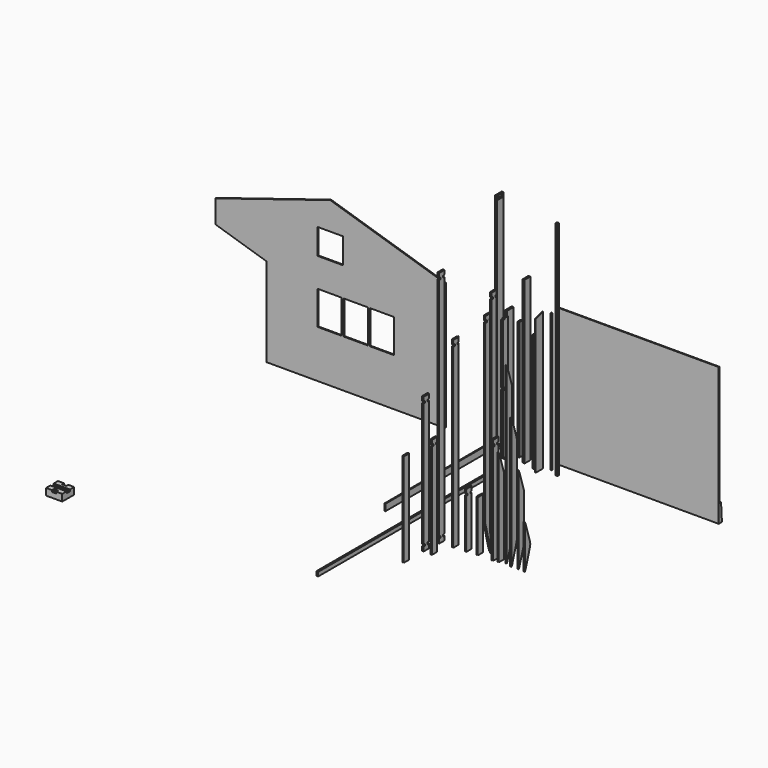
from build123d import *

# Parameters (mm, degrees)
F0_W      = 45
F0_H      = 195
F1_DEPTH  = 5255
F2_W      = 45
F2_H      = 195
F3_DEPTH  = 2945
F4_W      = 45
F4_H      = 145
F5_DEPTH  = 2914
F7_DEPTH  = 25
F8_W      = 3
F8_H      = 3
F9_DEPTH  = 5555
F10_W     = 45
F10_H     = 95
F11_DEPTH = 2800
F12_W     = 45
F12_H     = 170
F13_DEPTH = 3800
F14_W     = 45
F14_H     = 95
F15_DEPTH = 2768
F16_W     = 22
F16_H     = 220
F17_DEPTH = 3333
F19_DEPTH = 25
F20_W     = 3800
F20_H     = 19
F21_DEPTH = 3245
F22_W     = 25
F22_H     = 36
F23_DEPTH = 3245
F25_DEPTH = 25
F26_W     = 45
F26_H     = 45
F27_DEPTH = 5222
F29_DEPTH = 2956
F30_W     = 570
F30_H     = 150
F30_H_2   = 157
F30_H_3   = 483
F30_W_2   = 1200
F30_H_4   = 1603
F30_W_3   = 600
F30_H_5   = 600
F31_DEPTH = 25
F32_W     = 45
F32_H     = 95
F33_DEPTH = 5312
F36_DEPTH = 5600
F37_W     = 26
F37_H     = 43
F37_W_2   = 24
F37_W_3   = 31
F38_DEPTH = 55
F40_DEPTH = 3200
F41_W     = 31
F41_H     = 43
F41_W_2   = 24
F42_DEPTH = 55
F44_DEPTH = 4300
F45_W     = 31
F45_H     = 43
F45_W_2   = 24
F46_DEPTH = 55
F48_DEPTH = 1300
F49_W     = 31
F49_H     = 43
F49_W_2   = 24
F50_DEPTH = 55
F52_DEPTH = 1200
F54_DEPTH = 4980
F55_W     = 31
F55_H     = 43
F55_W_2   = 24
F56_DEPTH = 55
F58_DEPTH = 5493
F59_W     = 24
F59_H     = 43
F59_W_2   = 31
F60_DEPTH = 55
F62_DEPTH = 2500
F63_W     = 31
F63_H     = 43
F63_W_2   = 24
F64_DEPTH = 55
F66_DEPTH = 2271
F68_DEPTH = 55
F70_DEPTH = 4116
F72_DEPTH = 55
F74_DEPTH = 3088
F76_DEPTH = 55
F78_DEPTH = 2061
F80_DEPTH = 55
F82_DEPTH = 1034
F84_DEPTH = 55
F86_DEPTH = 2380
F87_W     = 31
F87_H     = 43
F87_W_2   = 24
F88_DEPTH = 55
F90_DEPTH = 2200
F91_W     = 37
F91_H     = 28.5
F91_H_2   = 45
F92_DEPTH = 55
F93_W     = 160
F93_H     = 45
F94_DEPTH = 55
F95_W     = 380
F95_H     = 350
F96_DEPTH = 160
F97_W     = 100
F97_H     = 52.8565406799
F97_W_2   = 380
F97_H_2   = 100
F97_H_3   = 60
F98_DEPTH = 40


with BuildPart() as f1:
    # F0 (on Top) → F1 (new body)
    with BuildSketch(Plane.XY):
        with Locations((-152.0553147793, 141.164868921)):
            Rectangle(F0_W, F0_H)
    extrude(amount=F1_DEPTH)

    # F93 (on face) → F94 (cut)
    with BuildSketch(Plane(origin=(-174.5553147793, 0, 0), x_dir=(0, -1, 0), z_dir=(-1, 0, 0))):
        with Locations((-128.664868921, 5187.5)):
            Rectangle(F93_W, F93_H)
        with Locations((-128.664868921, 67.5)):
            Rectangle(F93_W, F93_H)
    extrude(amount=-F94_DEPTH, mode=Mode.SUBTRACT)


with BuildPart() as f3:
    # F2 (on Top) → F3 (new body)
    with BuildSketch(Plane.XY):
        with Locations((71.8463295698, 157.7900274098)):
            Rectangle(F2_W, F2_H)
    extrude(amount=F3_DEPTH)


with BuildPart() as f5:
    # F4 (on Top) → F5 (new body)
    with BuildSketch(Plane.XY):
        with Locations((180.3632593155, -119.3333619833)):
            Rectangle(F4_W, F4_H)
    extrude(amount=F5_DEPTH)

    # F91 (on face) → F92 (cut)
    with BuildSketch(Plane.YZ.offset(202.8632593155)):
        with Locations((-173.3333619833, 2899.75)):
            Rectangle(F91_W, F91_H)
        with Locations((-173.3333619833, 1457)):
            Rectangle(F91_W, F91_H_2)
        with Locations((-173.3333619833, 14.25)):
            Rectangle(F91_W, F91_H)
    extrude(amount=-F92_DEPTH, mode=Mode.SUBTRACT)


with BuildPart() as f7:
    # F6 (on Front) → F7 (new body)
    with BuildSketch(Plane.XZ):
        Polygon((-6695.0071442492, 99.9302640557), (-1295.0071442492, 99.9302640557), (-1295.0071442492, 3099.9302640557), (-1339.0071442492, 3113.6347379577), (-1389.5608728424, 2951.3254020422), (-1432.52510882, 2964.7072713757), (-1381.9713802268, 3127.0166072912), (-3995.0071442492, 3940.886617132), (-6695.0071442492, 3099.9302640557), align=None)
    extrude(amount=F7_DEPTH)

    # F8 (on face) → F9 (cut)
    with BuildSketch(Plane(origin=(-6695.0071442492, 0, 0), x_dir=(0, -1, 0), z_dir=(-1, 0, 0))):
        with Locations((1.5, 261.4302640557)):
            Rectangle(F8_W, F8_H)
        with Locations((1.5, 421.4302640557)):
            Rectangle(F8_W, F8_H)
        with Locations((1.5, 741.4302640557)):
            Rectangle(F8_W, F8_H)
        with Locations((1.5, 901.4302640557)):
            Rectangle(F8_W, F8_H)
        with Locations((1.5, 1061.4302640557)):
            Rectangle(F8_W, F8_H)
        with Locations((1.5, 1221.4302640557)):
            Rectangle(F8_W, F8_H)
        with Locations((1.5, 1381.4302640557)):
            Rectangle(F8_W, F8_H)
        with Locations((1.5, 1541.4302640557)):
            Rectangle(F8_W, F8_H)
        with Locations((1.5, 1701.4302640557)):
            Rectangle(F8_W, F8_H)
        with Locations((1.5, 1861.4302640557)):
            Rectangle(F8_W, F8_H)
        with Locations((1.5, 2021.4302640557)):
            Rectangle(F8_W, F8_H)
        with Locations((1.5, 581.4302640557)):
            Rectangle(F8_W, F8_H)
        with Locations((1.5, 2181.4302640557)):
            Rectangle(F8_W, F8_H)
        with Locations((1.5, 2341.4302640557)):
            Rectangle(F8_W, F8_H)
        with Locations((1.5, 2501.4302640557)):
            Rectangle(F8_W, F8_H)
        with Locations((1.5, 2661.4302640557)):
            Rectangle(F8_W, F8_H)
        with Locations((1.5, 2821.4302640557)):
            Rectangle(F8_W, F8_H)
        with Locations((1.5, 2981.4302640557)):
            Rectangle(F8_W, F8_H)
        with Locations((1.5, 3141.4302640557)):
            Rectangle(F8_W, F8_H)
        with Locations((1.5, 3301.4302640557)):
            Rectangle(F8_W, F8_H)
        with Locations((1.5, 3461.4302640557)):
            Rectangle(F8_W, F8_H)
        with Locations((1.5, 3621.4302640557)):
            Rectangle(F8_W, F8_H)
        with Locations((1.5, 3781.4302640557)):
            Rectangle(F8_W, F8_H)
        with Locations((1.5, 3941.4302640557)):
            Rectangle(F8_W, F8_H)
        with Locations((1.5, 4101.4302640557)):
            Rectangle(F8_W, F8_H)
    extrude(amount=-F9_DEPTH, mode=Mode.SUBTRACT)

    # F30 (on face) → F31 (cut)
    with BuildSketch(Plane(origin=(0, 0, 0), x_dir=(-1, 0, 0), z_dir=(0, 1, 0))):
        with Locations((4010.0071442492, 1934.9302640557)):
            Rectangle(F30_W, F30_H)
        with Locations((4010.0071442492, 1781.4302640557)):
            Rectangle(F30_W, F30_H_2)
        with Locations((3395.0071442492, 1934.9302640557)):
            Rectangle(F30_W, F30_H)
        with Locations((4010.0071442492, 1461.4302640557)):
            Rectangle(F30_W, F30_H_3)
        with Locations((6095.0071442492, 1781.4302640557)):
            Rectangle(F30_W_2, F30_H_2)
        Polygon((5495.0071442492, 2187.9302640557), (5495.0071442492, 1859.9302640557), (6695.0071442492, 1859.9302640557), (6695.0071442492, 2561.6886432007), align=None)
        with Locations((3395.0071442492, 1781.4302640557)):
            Rectangle(F30_W, F30_H_2)
        with Locations((6095.0071442492, 901.4302640557)):
            Rectangle(F30_W_2, F30_H_4)
        with Locations((2780.0071442492, 1934.9302640557)):
            Rectangle(F30_W, F30_H)
        with Locations((3395.0071442492, 1461.4302640557)):
            Rectangle(F30_W, F30_H_3)
        with Locations((2780.0071442492, 1781.4302640557)):
            Rectangle(F30_W, F30_H_2)
        with Locations((2780.0071442492, 1461.4302640557)):
            Rectangle(F30_W, F30_H_3)
        with Locations((3995.0071442492, 2989.9302640557)):
            Rectangle(F30_W_3, F30_H_5)
    extrude(amount=-F31_DEPTH, mode=Mode.SUBTRACT)


with BuildPart() as f11:
    # F10 (on Top) → F11 (new body)
    with BuildSketch(Plane.XY):
        with Locations((358.6191916466, 109.5414018631)):
            Rectangle(F10_W, F10_H)
    extrude(amount=F11_DEPTH)


with BuildPart() as f13:
    # F12 (on Top) → F13 (new body)
    with BuildSketch(Plane.XY):
        with Locations((580.7736301422, 26.5171183646)):
            Rectangle(F12_W, F12_H)
    extrude(amount=F13_DEPTH)


with BuildPart() as f15:
    # F14 (on Top) → F15 (new body)
    with BuildSketch(Plane.XY):
        with Locations((861.2215881348, -79.6096616983)):
            Rectangle(F14_W, F14_H)
    extrude(amount=F15_DEPTH)


with BuildPart() as f17:
    # F16 (on Top) → F17 (new body)
    with BuildSketch(Plane.XY):
        with Locations((982.1879491806, -110)):
            Rectangle(F16_W, F16_H)
    extrude(amount=F17_DEPTH)

    # F18 (on face) → F19 (cut)
    with BuildSketch(Plane.YZ.offset(993.1879491806)):
        Polygon((-220, 3264.4776304901), (0, 3333), (-220, 3333), align=None)
        Polygon((0, 3245.66), (0, 3333), (-220, 3264.4776304901), (-220, 3177.1376304901), align=None)
    extrude(amount=-F19_DEPTH, mode=Mode.SUBTRACT)


with BuildPart() as f21:
    # F20 (on Top) → F21 (new body)
    with BuildSketch(Plane.XY):
        with Locations((2986.4132642746, 300.9606630802)):
            Rectangle(F20_W, F20_H)
    extrude(amount=F21_DEPTH)


with BuildPart() as f23:
    # F22 (on Top) → F23 (new body)
    with BuildSketch(Plane.XY):
        with Locations((1146.2202548981, 50.4518755078)):
            Rectangle(F22_W, F22_H)
    extrude(amount=F23_DEPTH)


with BuildPart() as f25:
    # F24 (on face) → F25 (new body)
    with BuildSketch(Plane.YZ.offset(4886.4132642746)):
        Polygon((385.4606630802, 0), (360.4606630802, 419.255292155), (310.4606630802, 419.255292155), (310.4606630802, 0), align=None)
    extrude(amount=-F25_DEPTH)


with BuildPart() as f27:
    # F26 (on Top) → F27 (new body)
    with BuildSketch(Plane.XY):
        with Locations((1366.4702558517, -54.2847523093)):
            Rectangle(F26_W, F26_H)
    extrude(amount=F27_DEPTH)


with BuildPart() as f29:
    # F28 (on Front) → F29 (new body)
    with BuildSketch(Plane.XZ):
        with BuildLine():
            Line((-358.2668054104, 33.0118125677), (-375.2668054104, 33.0118125677))
            Line((-375.2668054104, 33.0118125677), (-375.2668054104, -126.9881874323))
            Line((-375.2668054104, -126.9881874323), (-358.2668054104, -126.9881874323))
            ThreePointArc((-358.2668054104, -126.9881874323), (-354.7312715045, -125.5237213382), (-353.2668054104, -121.9881874323))
            Line((-353.2668054104, -121.9881874323), (-353.2668054104, 28.0118125677))
            ThreePointArc((-353.2668054104, 28.0118125677), (-354.7312715045, 31.5473464736), (-358.2668054104, 33.0118125677))
        make_face()
    extrude(amount=F29_DEPTH)


with BuildPart() as f33:
    # F32 (on Front) → F33 (new body)
    with BuildSketch(Plane.XZ):
        with Locations((-70.3556007147, -368.9510369301)):
            Rectangle(F32_W, F32_H)
    extrude(amount=F33_DEPTH)


with BuildPart() as f36:
    # F35 (on face) → F36 (new body)
    with BuildSketch(Plane.XY):
        with BuildLine():
            Line((1341.7238235474, -3371.5739750846), (1332.4738235474, -3371.5739750846))
            Line((1332.4738235474, -3371.5739750846), (1326.4738235474, -3387.5739750846))
            Line((1326.4738235474, -3387.5739750846), (1326.4738235474, -3515.5739750846))
            Line((1326.4738235474, -3515.5739750846), (1332.4738235474, -3531.5739750846))
            Line((1332.4738235474, -3531.5739750846), (1340.5536906658, -3531.5739750846))
            ThreePointArc((1340.5536906658, -3531.5739750846), (1341.2308001548, -3531.3098573713), (1341.550236424, -3530.6570205645))
            Line((1341.550236424, -3530.6570205645), (1342.3974106707, -3520.4909296048))
            ThreePointArc((1342.3974106707, -3520.4909296048), (1342.7168469399, -3519.8380927979), (1343.3939564289, -3519.5739750846))
            Line((1343.3939564289, -3519.5739750846), (1352.5536906658, -3519.5739750846))
            ThreePointArc((1352.5536906658, -3519.5739750846), (1353.2308001548, -3519.8380927979), (1353.550236424, -3520.4909296048))
            Line((1353.550236424, -3520.4909296048), (1354.3974106707, -3530.6570205645))
            ThreePointArc((1354.3974106707, -3530.6570205645), (1354.7168469399, -3531.3098573713), (1355.3939564289, -3531.5739750846))
            Line((1355.3939564289, -3531.5739750846), (1363.4738235474, -3531.5739750846))
            Line((1363.4738235474, -3531.5739750846), (1369.4738235474, -3515.5739750846))
            Line((1369.4738235474, -3515.5739750846), (1369.4738235474, -3387.5739750846))
            Line((1369.4738235474, -3387.5739750846), (1363.4738235474, -3371.5739750846))
            Line((1363.4738235474, -3371.5739750846), (1354.2238235474, -3371.5739750846))
            Line((1354.2238235474, -3371.5739750846), (1341.7238235474, -3371.5739750846))
        make_face()
        with BuildLine():
            Line((1342.6376148895, -3361.979165992), (1341.7238235474, -3371.5739750846))
            Line((1341.7238235474, -3371.5739750846), (1354.2238235474, -3371.5739750846))
            Line((1354.2238235474, -3371.5739750846), (1353.3100322052, -3361.979165992))
            ThreePointArc((1353.3100322052, -3361.979165992), (1352.9872888814, -3361.3341071597), (1352.3145367326, -3361.0739750846))
            Line((1352.3145367326, -3361.0739750846), (1343.6331103621, -3361.0739750846))
            ThreePointArc((1343.6331103621, -3361.0739750846), (1342.9603582133, -3361.3341071597), (1342.6376148895, -3361.979165992))
        make_face()
    extrude(amount=F36_DEPTH)

    # F37 (on face) → F38 (cut)
    with BuildSketch(Plane.YZ.offset(1369.4738235474)):
        with Locations((-3528.5739750846, 5478.5)):
            Rectangle(F37_W, F37_H)
        with Locations((-3503.5739750846, 5478.5)):
            Rectangle(F37_W_2, F37_H)
        with Locations((-3399.5739750846, 5478.5)):
            Rectangle(F37_W_2, F37_H)
        with Locations((-3372.0739750846, 5478.5)):
            Rectangle(F37_W_3, F37_H)
        with Locations((-3503.5739750846, 121.5)):
            Rectangle(F37_W_2, F37_H)
        with Locations((-3528.5739750846, 121.5)):
            Rectangle(F37_W, F37_H)
        with Locations((-3399.5739750846, 121.5)):
            Rectangle(F37_W_2, F37_H)
        with Locations((-3372.0739750846, 121.5)):
            Rectangle(F37_W_3, F37_H)
    extrude(amount=-F38_DEPTH, mode=Mode.SUBTRACT)


with BuildPart() as f40:
    # F39 (on face) → F40 (new body)
    with BuildSketch(Plane.XY):
        with BuildLine():
            Line((1314.3787622452, -3790.5488514884), (1305.1287622452, -3790.5488514884))
            Line((1305.1287622452, -3790.5488514884), (1299.1287622452, -3806.5488514884))
            Line((1299.1287622452, -3806.5488514884), (1299.1287622452, -3934.5488514884))
            Line((1299.1287622452, -3934.5488514884), (1305.1287622452, -3950.5488514884))
            Line((1305.1287622452, -3950.5488514884), (1313.2086293636, -3950.5488514884))
            ThreePointArc((1313.2086293636, -3950.5488514884), (1313.8857388526, -3950.2847337751), (1314.2051751219, -3949.6318969683))
            Line((1314.2051751219, -3949.6318969683), (1315.0523493685, -3939.4658060086))
            ThreePointArc((1315.0523493685, -3939.4658060086), (1315.3717856378, -3938.8129692017), (1316.0488951267, -3938.5488514884))
            Line((1316.0488951267, -3938.5488514884), (1325.2086293636, -3938.5488514884))
            ThreePointArc((1325.2086293636, -3938.5488514884), (1325.8857388526, -3938.8129692017), (1326.2051751219, -3939.4658060086))
            Line((1326.2051751219, -3939.4658060086), (1327.0523493685, -3949.6318969683))
            ThreePointArc((1327.0523493685, -3949.6318969683), (1327.3717856378, -3950.2847337751), (1328.0488951267, -3950.5488514884))
            Line((1328.0488951267, -3950.5488514884), (1336.1287622452, -3950.5488514884))
            Line((1336.1287622452, -3950.5488514884), (1342.1287622452, -3934.5488514884))
            Line((1342.1287622452, -3934.5488514884), (1342.1287622452, -3806.5488514884))
            Line((1342.1287622452, -3806.5488514884), (1336.1287622452, -3790.5488514884))
            Line((1336.1287622452, -3790.5488514884), (1326.8787622452, -3790.5488514884))
            Line((1326.8787622452, -3790.5488514884), (1314.3787622452, -3790.5488514884))
        make_face()
        with BuildLine():
            Line((1315.2925535873, -3780.9540423958), (1314.3787622452, -3790.5488514884))
            Line((1314.3787622452, -3790.5488514884), (1326.8787622452, -3790.5488514884))
            Line((1326.8787622452, -3790.5488514884), (1325.964970903, -3780.9540423958))
            ThreePointArc((1325.964970903, -3780.9540423958), (1325.6422275792, -3780.3089835635), (1324.9694754304, -3780.0488514884))
            Line((1324.9694754304, -3780.0488514884), (1316.2880490599, -3780.0488514884))
            ThreePointArc((1316.2880490599, -3780.0488514884), (1315.6152969111, -3780.3089835635), (1315.2925535873, -3780.9540423958))
        make_face()
    extrude(amount=F40_DEPTH)

    # F41 (on face) → F42 (cut)
    with BuildSketch(Plane.YZ.offset(1342.1287622452)):
        with Locations((-3791.0488514884, 3078.5)):
            Rectangle(F41_W, F41_H)
        with Locations((-3818.5488514884, 3078.5)):
            Rectangle(F41_W_2, F41_H)
        with Locations((-3922.5488514884, 3078.5)):
            Rectangle(F41_W_2, F41_H)
        with Locations((-3950.0488514884, 3078.5)):
            Rectangle(F41_W, F41_H)
        with Locations((-3791.0488514884, 121.5)):
            Rectangle(F41_W, F41_H)
        with Locations((-3818.5488514884, 121.5)):
            Rectangle(F41_W_2, F41_H)
        with Locations((-3950.0488514884, 121.5)):
            Rectangle(F41_W, F41_H)
        with Locations((-3922.5488514884, 121.5)):
            Rectangle(F41_W_2, F41_H)
    extrude(amount=-F42_DEPTH, mode=Mode.SUBTRACT)


with BuildPart() as f44:
    # F43 (on face) → F44 (new body)
    with BuildSketch(Plane.XY):
        with BuildLine():
            Line((1648.11398983, -3331.4161801322), (1638.86398983, -3331.4161801322))
            Line((1638.86398983, -3331.4161801322), (1632.86398983, -3347.4161801322))
            Line((1632.86398983, -3347.4161801322), (1632.86398983, -3475.4161801322))
            Line((1632.86398983, -3475.4161801322), (1638.86398983, -3491.4161801322))
            Line((1638.86398983, -3491.4161801322), (1646.9438569485, -3491.4161801322))
            ThreePointArc((1646.9438569485, -3491.4161801322), (1647.6209664374, -3491.1520624189), (1647.9404027067, -3490.4992256121))
            Line((1647.9404027067, -3490.4992256121), (1648.7875769533, -3480.3331346524))
            ThreePointArc((1648.7875769533, -3480.3331346524), (1649.1070132226, -3479.6802978455), (1649.7841227116, -3479.4161801322))
            Line((1649.7841227116, -3479.4161801322), (1658.9438569485, -3479.4161801322))
            ThreePointArc((1658.9438569485, -3479.4161801322), (1659.6209664374, -3479.6802978455), (1659.9404027067, -3480.3331346524))
            Line((1659.9404027067, -3480.3331346524), (1660.7875769533, -3490.4992256121))
            ThreePointArc((1660.7875769533, -3490.4992256121), (1661.1070132226, -3491.1520624189), (1661.7841227116, -3491.4161801322))
            Line((1661.7841227116, -3491.4161801322), (1669.86398983, -3491.4161801322))
            Line((1669.86398983, -3491.4161801322), (1675.86398983, -3475.4161801322))
            Line((1675.86398983, -3475.4161801322), (1675.86398983, -3347.4161801322))
            Line((1675.86398983, -3347.4161801322), (1669.86398983, -3331.4161801322))
            Line((1669.86398983, -3331.4161801322), (1660.61398983, -3331.4161801322))
            Line((1660.61398983, -3331.4161801322), (1648.11398983, -3331.4161801322))
        make_face()
        with BuildLine():
            Line((1649.0277811722, -3321.8213710396), (1648.11398983, -3331.4161801322))
            Line((1648.11398983, -3331.4161801322), (1660.61398983, -3331.4161801322))
            Line((1660.61398983, -3331.4161801322), (1659.7001984879, -3321.8213710396))
            ThreePointArc((1659.7001984879, -3321.8213710396), (1659.377455164, -3321.1763122073), (1658.7047030153, -3320.9161801322))
            Line((1658.7047030153, -3320.9161801322), (1650.0232766448, -3320.9161801322))
            ThreePointArc((1650.0232766448, -3320.9161801322), (1649.350524496, -3321.1763122073), (1649.0277811722, -3321.8213710396))
        make_face()
    extrude(amount=F44_DEPTH)

    # F45 (on face) → F46 (cut)
    with BuildSketch(Plane.YZ.offset(1675.86398983)):
        with Locations((-3331.9161801322, 4178.5)):
            Rectangle(F45_W, F45_H)
        with Locations((-3359.4161801322, 4178.5)):
            Rectangle(F45_W_2, F45_H)
        with Locations((-3463.4161801322, 4178.5)):
            Rectangle(F45_W_2, F45_H)
        with Locations((-3490.9161801322, 4178.5)):
            Rectangle(F45_W, F45_H)
    extrude(amount=-F46_DEPTH, mode=Mode.SUBTRACT)


with BuildPart() as f48:
    # F47 (on face) → F48 (new body)
    with BuildSketch(Plane.XY):
        with BuildLine():
            Line((1937.5608205795, -3313.5357403739), (1928.3108205795, -3313.5357403739))
            Line((1928.3108205795, -3313.5357403739), (1922.3108205795, -3329.5357403739))
            Line((1922.3108205795, -3329.5357403739), (1922.3108205795, -3457.5357403739))
            Line((1922.3108205795, -3457.5357403739), (1928.3108205795, -3473.5357403739))
            Line((1928.3108205795, -3473.5357403739), (1936.390687698, -3473.5357403739))
            ThreePointArc((1936.390687698, -3473.5357403739), (1937.0677971869, -3473.2716226606), (1937.3872334562, -3472.6187858538))
            Line((1937.3872334562, -3472.6187858538), (1938.2344077028, -3462.4526948941))
            ThreePointArc((1938.2344077028, -3462.4526948941), (1938.5538439721, -3461.7998580872), (1939.2309534611, -3461.5357403739))
            Line((1939.2309534611, -3461.5357403739), (1948.390687698, -3461.5357403739))
            ThreePointArc((1948.390687698, -3461.5357403739), (1949.0677971869, -3461.7998580872), (1949.3872334562, -3462.4526948941))
            Line((1949.3872334562, -3462.4526948941), (1950.2344077028, -3472.6187858538))
            ThreePointArc((1950.2344077028, -3472.6187858538), (1950.5538439721, -3473.2716226606), (1951.2309534611, -3473.5357403739))
            Line((1951.2309534611, -3473.5357403739), (1959.3108205795, -3473.5357403739))
            Line((1959.3108205795, -3473.5357403739), (1965.3108205795, -3457.5357403739))
            Line((1965.3108205795, -3457.5357403739), (1965.3108205795, -3329.5357403739))
            Line((1965.3108205795, -3329.5357403739), (1959.3108205795, -3313.5357403739))
            Line((1959.3108205795, -3313.5357403739), (1950.0608205795, -3313.5357403739))
            Line((1950.0608205795, -3313.5357403739), (1937.5608205795, -3313.5357403739))
        make_face()
        with BuildLine():
            Line((1938.4746119217, -3303.9409312813), (1937.5608205795, -3313.5357403739))
            Line((1937.5608205795, -3313.5357403739), (1950.0608205795, -3313.5357403739))
            Line((1950.0608205795, -3313.5357403739), (1949.1470292374, -3303.9409312813))
            ThreePointArc((1949.1470292374, -3303.9409312813), (1948.8242859136, -3303.295872449), (1948.1515337648, -3303.0357403739))
            Line((1948.1515337648, -3303.0357403739), (1939.4701073943, -3303.0357403739))
            ThreePointArc((1939.4701073943, -3303.0357403739), (1938.7973552455, -3303.295872449), (1938.4746119217, -3303.9409312813))
        make_face()
    extrude(amount=F48_DEPTH)

    # F49 (on face) → F50 (cut)
    with BuildSketch(Plane.YZ.offset(1965.3108205795)):
        with Locations((-3314.0357403739, 1178.5)):
            Rectangle(F49_W, F49_H)
        with Locations((-3341.5357403739, 1178.5)):
            Rectangle(F49_W_2, F49_H)
        with Locations((-3445.5357403739, 1178.5)):
            Rectangle(F49_W_2, F49_H)
        with Locations((-3473.0357403739, 1178.5)):
            Rectangle(F49_W, F49_H)
    extrude(amount=-F50_DEPTH, mode=Mode.SUBTRACT)


with BuildPart() as f52:
    # F51 (on face) → F52 (new body)
    with BuildSketch(Plane.XY):
        with BuildLine():
            Line((2187.5275611877, -3287.7691292747), (2178.2775611877, -3287.7691292747))
            Line((2178.2775611877, -3287.7691292747), (2172.2775611877, -3303.7691292747))
            Line((2172.2775611877, -3303.7691292747), (2172.2775611877, -3431.7691292747))
            Line((2172.2775611877, -3431.7691292747), (2178.2775611877, -3447.7691292747))
            Line((2178.2775611877, -3447.7691292747), (2186.3574283062, -3447.7691292747))
            ThreePointArc((2186.3574283062, -3447.7691292747), (2187.0345377952, -3447.5050115614), (2187.3539740644, -3446.8521747545))
            Line((2187.3539740644, -3446.8521747545), (2188.2011483111, -3436.6860837948))
            ThreePointArc((2188.2011483111, -3436.6860837948), (2188.5205845803, -3436.0332469879), (2189.1976940693, -3435.7691292747))
            Line((2189.1976940693, -3435.7691292747), (2198.3574283062, -3435.7691292747))
            ThreePointArc((2198.3574283062, -3435.7691292747), (2199.0345377952, -3436.0332469879), (2199.3539740644, -3436.6860837948))
            Line((2199.3539740644, -3436.6860837948), (2200.2011483111, -3446.8521747545))
            ThreePointArc((2200.2011483111, -3446.8521747545), (2200.5205845803, -3447.5050115614), (2201.1976940693, -3447.7691292747))
            Line((2201.1976940693, -3447.7691292747), (2209.2775611877, -3447.7691292747))
            Line((2209.2775611877, -3447.7691292747), (2215.2775611877, -3431.7691292747))
            Line((2215.2775611877, -3431.7691292747), (2215.2775611877, -3303.7691292747))
            Line((2215.2775611877, -3303.7691292747), (2209.2775611877, -3287.7691292747))
            Line((2209.2775611877, -3287.7691292747), (2200.0275611877, -3287.7691292747))
            Line((2200.0275611877, -3287.7691292747), (2187.5275611877, -3287.7691292747))
        make_face()
        with BuildLine():
            Line((2188.4413525299, -3278.174320182), (2187.5275611877, -3287.7691292747))
            Line((2187.5275611877, -3287.7691292747), (2200.0275611877, -3287.7691292747))
            Line((2200.0275611877, -3287.7691292747), (2199.1137698456, -3278.174320182))
            ThreePointArc((2199.1137698456, -3278.174320182), (2198.7910265218, -3277.5292613498), (2198.118274373, -3277.2691292747))
            Line((2198.118274373, -3277.2691292747), (2189.4368480025, -3277.2691292747))
            ThreePointArc((2189.4368480025, -3277.2691292747), (2188.7640958537, -3277.5292613498), (2188.4413525299, -3278.174320182))
        make_face()
    extrude(amount=F52_DEPTH)


with BuildPart() as f54:
    # F53 (on face) → F54 (new body)
    with BuildSketch(Plane.XY):
        with BuildLine():
            Line((2329.9156665802, -3244.56625223), (2320.6656665802, -3244.56625223))
            Line((2320.6656665802, -3244.56625223), (2314.6656665802, -3260.56625223))
            Line((2314.6656665802, -3260.56625223), (2314.6656665802, -3388.56625223))
            Line((2314.6656665802, -3388.56625223), (2320.6656665802, -3404.56625223))
            Line((2320.6656665802, -3404.56625223), (2328.7455336986, -3404.56625223))
            ThreePointArc((2328.7455336986, -3404.56625223), (2329.4226431876, -3404.3021345167), (2329.7420794569, -3403.6492977098))
            Line((2329.7420794569, -3403.6492977098), (2330.5892537035, -3393.4832067501))
            ThreePointArc((2330.5892537035, -3393.4832067501), (2330.9086899728, -3392.8303699433), (2331.5857994618, -3392.56625223))
            Line((2331.5857994618, -3392.56625223), (2340.7455336986, -3392.56625223))
            ThreePointArc((2340.7455336986, -3392.56625223), (2341.4226431876, -3392.8303699433), (2341.7420794569, -3393.4832067501))
            Line((2341.7420794569, -3393.4832067501), (2342.5892537035, -3403.6492977098))
            ThreePointArc((2342.5892537035, -3403.6492977098), (2342.9086899728, -3404.3021345167), (2343.5857994618, -3404.56625223))
            Line((2343.5857994618, -3404.56625223), (2351.6656665802, -3404.56625223))
            Line((2351.6656665802, -3404.56625223), (2357.6656665802, -3388.56625223))
            Line((2357.6656665802, -3388.56625223), (2357.6656665802, -3260.56625223))
            Line((2357.6656665802, -3260.56625223), (2351.6656665802, -3244.56625223))
            Line((2351.6656665802, -3244.56625223), (2342.4156665802, -3244.56625223))
            Line((2342.4156665802, -3244.56625223), (2329.9156665802, -3244.56625223))
        make_face()
        with BuildLine():
            Line((2330.8294579224, -3234.9714431374), (2329.9156665802, -3244.56625223))
            Line((2329.9156665802, -3244.56625223), (2342.4156665802, -3244.56625223))
            Line((2342.4156665802, -3244.56625223), (2341.501875238, -3234.9714431374))
            ThreePointArc((2341.501875238, -3234.9714431374), (2341.1791319142, -3234.3263843051), (2340.5063797655, -3234.06625223))
            Line((2340.5063797655, -3234.06625223), (2331.8249533949, -3234.06625223))
            ThreePointArc((2331.8249533949, -3234.06625223), (2331.1522012462, -3234.3263843051), (2330.8294579224, -3234.9714431374))
        make_face()
    extrude(amount=F54_DEPTH)

    # F55 (on face) → F56 (cut)
    with BuildSketch(Plane.YZ.offset(2357.6656665802)):
        with Locations((-3245.06625223, 4858.5)):
            Rectangle(F55_W, F55_H)
        with Locations((-3376.56625223, 4858.5)):
            Rectangle(F55_W_2, F55_H)
        with Locations((-3404.06625223, 4858.5)):
            Rectangle(F55_W, F55_H)
        with Locations((-3272.56625223, 4858.5)):
            Rectangle(F55_W_2, F55_H)
        Polygon((-3260.56625223, 0), (-3260.56625223, 102.6551723062), (-3388.56625223, 616.0351317988), (-3388.56625223, 0), align=None)
        Polygon((-3175.0889188828, -240.1756865324), (-3260.56625223, 102.6551723062), (-3260.56625223, 0), (-3388.56625223, 0), (-3388.56625223, 616.0351317988), (-3443.864144894, 837.8228653603), (-3443.864144894, -302.3062239952), align=None)
    extrude(amount=-F56_DEPTH, mode=Mode.SUBTRACT)


with BuildPart() as f58:
    # F57 (on face) → F58 (new body)
    with BuildSketch(Plane.XY):
        with BuildLine():
            Line((2454.8987388611, -3221.3349843009), (2445.6487388611, -3221.3349843009))
            Line((2445.6487388611, -3221.3349843009), (2439.6487388611, -3237.3349843009))
            Line((2439.6487388611, -3237.3349843009), (2439.6487388611, -3365.3349843009))
            Line((2439.6487388611, -3365.3349843009), (2445.6487388611, -3381.3349843009))
            Line((2445.6487388611, -3381.3349843009), (2453.7286059795, -3381.3349843009))
            ThreePointArc((2453.7286059795, -3381.3349843009), (2454.4057154685, -3381.0708665876), (2454.7251517378, -3380.4180297808))
            Line((2454.7251517378, -3380.4180297808), (2455.5723259844, -3370.2519388211))
            ThreePointArc((2455.5723259844, -3370.2519388211), (2455.8917622537, -3369.5991020142), (2456.5688717427, -3369.3349843009))
            Line((2456.5688717427, -3369.3349843009), (2465.7286059795, -3369.3349843009))
            ThreePointArc((2465.7286059795, -3369.3349843009), (2466.4057154685, -3369.5991020142), (2466.7251517378, -3370.2519388211))
            Line((2466.7251517378, -3370.2519388211), (2467.5723259844, -3380.4180297808))
            ThreePointArc((2467.5723259844, -3380.4180297808), (2467.8917622537, -3381.0708665876), (2468.5688717426, -3381.3349843009))
            Line((2468.5688717426, -3381.3349843009), (2476.6487388611, -3381.3349843009))
            Line((2476.6487388611, -3381.3349843009), (2482.6487388611, -3365.3349843009))
            Line((2482.6487388611, -3365.3349843009), (2482.6487388611, -3237.3349843009))
            Line((2482.6487388611, -3237.3349843009), (2476.6487388611, -3221.3349843009))
            Line((2476.6487388611, -3221.3349843009), (2467.3987388611, -3221.3349843009))
            Line((2467.3987388611, -3221.3349843009), (2454.8987388611, -3221.3349843009))
        make_face()
        with BuildLine():
            Line((2455.8125302032, -3211.7401752083), (2454.8987388611, -3221.3349843009))
            Line((2454.8987388611, -3221.3349843009), (2467.3987388611, -3221.3349843009))
            Line((2467.3987388611, -3221.3349843009), (2466.4849475189, -3211.7401752083))
            ThreePointArc((2466.4849475189, -3211.7401752083), (2466.1622041951, -3211.095116376), (2465.4894520463, -3210.8349843009))
            Line((2465.4894520463, -3210.8349843009), (2456.8080256758, -3210.8349843009))
            ThreePointArc((2456.8080256758, -3210.8349843009), (2456.1352735271, -3211.095116376), (2455.8125302032, -3211.7401752083))
        make_face()
    extrude(amount=F58_DEPTH)

    # F59 (on face) → F60 (cut)
    with BuildSketch(Plane.YZ.offset(2482.6487388611)):
        Polygon((-3237.3349843009, 0), (-3237.3349843009, 82.1754711732), (-3365.3349843009, 493.136157463), (-3365.3349843009, 0), align=None)
        Polygon((-3127.8158909651, -269.4498550702), (-3237.3349843009, 82.1754711732), (-3237.3349843009, 0), (-3365.3349843009, 0), (-3365.3349843009, 493.136157463), (-3523.9308768201, 1002.3289452164), (-3523.9308768201, -321.5949704082), align=None)
        with Locations((-3249.3349843009, 5371.5)):
            Rectangle(F59_W, F59_H)
        with Locations((-3221.8349843009, 5371.5)):
            Rectangle(F59_W_2, F59_H)
        with Locations((-3380.8349843009, 5371.5)):
            Rectangle(F59_W_2, F59_H)
        with Locations((-3353.3349843009, 5371.5)):
            Rectangle(F59_W, F59_H)
    extrude(amount=-F60_DEPTH, mode=Mode.SUBTRACT)


with BuildPart() as f62:
    # F61 (on face) → F62 (new body)
    with BuildSketch(Plane.XY):
        with BuildLine():
            Line((2541.8647766113, -3282.0468449577), (2532.6147766113, -3282.0468449577))
            Line((2532.6147766113, -3282.0468449577), (2526.6147766113, -3298.0468449577))
            Line((2526.6147766113, -3298.0468449577), (2526.6147766113, -3426.0468449577))
            Line((2526.6147766113, -3426.0468449577), (2532.6147766113, -3442.0468449577))
            Line((2532.6147766113, -3442.0468449577), (2540.6946437298, -3442.0468449577))
            ThreePointArc((2540.6946437298, -3442.0468449577), (2541.3717532187, -3441.7827272444), (2541.691189488, -3441.1298904375))
            Line((2541.691189488, -3441.1298904375), (2542.5383637346, -3430.9637994778))
            ThreePointArc((2542.5383637346, -3430.9637994778), (2542.8578000039, -3430.3109626709), (2543.5349094929, -3430.0468449577))
            Line((2543.5349094929, -3430.0468449577), (2552.6946437298, -3430.0468449577))
            ThreePointArc((2552.6946437298, -3430.0468449577), (2553.3717532187, -3430.3109626709), (2553.691189488, -3430.9637994778))
            Line((2553.691189488, -3430.9637994778), (2554.5383637346, -3441.1298904375))
            ThreePointArc((2554.5383637346, -3441.1298904375), (2554.8578000039, -3441.7827272444), (2555.5349094929, -3442.0468449577))
            Line((2555.5349094929, -3442.0468449577), (2563.6147766113, -3442.0468449577))
            Line((2563.6147766113, -3442.0468449577), (2569.6147766113, -3426.0468449577))
            Line((2569.6147766113, -3426.0468449577), (2569.6147766113, -3298.0468449577))
            Line((2569.6147766113, -3298.0468449577), (2563.6147766113, -3282.0468449577))
            Line((2563.6147766113, -3282.0468449577), (2554.3647766113, -3282.0468449577))
            Line((2554.3647766113, -3282.0468449577), (2541.8647766113, -3282.0468449577))
        make_face()
        with BuildLine():
            Line((2542.7785679535, -3272.452035865), (2541.8647766113, -3282.0468449577))
            Line((2541.8647766113, -3282.0468449577), (2554.3647766113, -3282.0468449577))
            Line((2554.3647766113, -3282.0468449577), (2553.4509852692, -3272.452035865))
            ThreePointArc((2553.4509852692, -3272.452035865), (2553.1282419454, -3271.8069770327), (2552.4554897966, -3271.5468449577))
            Line((2552.4554897966, -3271.5468449577), (2543.7740634261, -3271.5468449577))
            ThreePointArc((2543.7740634261, -3271.5468449577), (2543.1013112773, -3271.8069770327), (2542.7785679535, -3272.452035865))
        make_face()
    extrude(amount=F62_DEPTH)

    # F63 (on face) → F64 (cut)
    with BuildSketch(Plane.YZ.offset(2569.6147766113)):
        with Locations((-3282.5468449577, 2378.5)):
            Rectangle(F63_W, F63_H)
        with Locations((-3310.0468449577, 2378.5)):
            Rectangle(F63_W_2, F63_H)
        with Locations((-3414.0468449577, 2378.5)):
            Rectangle(F63_W_2, F63_H)
        with Locations((-3441.5468449577, 2378.5)):
            Rectangle(F63_W, F63_H)
    extrude(amount=-F64_DEPTH, mode=Mode.SUBTRACT)


with BuildPart() as f66:
    # F65 (on face) → F66 (new body)
    with BuildSketch(Plane.XY):
        with BuildLine():
            Line((2661.9013786316, -3260.6926465018), (2652.6513786316, -3260.6926465018))
            Line((2652.6513786316, -3260.6926465018), (2646.6513786316, -3276.6926465018))
            Line((2646.6513786316, -3276.6926465018), (2646.6513786316, -3404.6926465018))
            Line((2646.6513786316, -3404.6926465018), (2652.6513786316, -3420.6926465018))
            Line((2652.6513786316, -3420.6926465018), (2660.73124575, -3420.6926465018))
            ThreePointArc((2660.73124575, -3420.6926465018), (2661.408355239, -3420.4285287886), (2661.7277915083, -3419.7756919817))
            Line((2661.7277915083, -3419.7756919817), (2662.5749657549, -3409.609601022))
            ThreePointArc((2662.5749657549, -3409.609601022), (2662.8944020242, -3408.9567642151), (2663.5715115132, -3408.6926465018))
            Line((2663.5715115132, -3408.6926465018), (2672.73124575, -3408.6926465018))
            ThreePointArc((2672.73124575, -3408.6926465018), (2673.408355239, -3408.9567642151), (2673.7277915083, -3409.609601022))
            Line((2673.7277915083, -3409.609601022), (2674.5749657549, -3419.7756919817))
            ThreePointArc((2674.5749657549, -3419.7756919817), (2674.8944020242, -3420.4285287886), (2675.5715115132, -3420.6926465018))
            Line((2675.5715115132, -3420.6926465018), (2683.6513786316, -3420.6926465018))
            Line((2683.6513786316, -3420.6926465018), (2689.6513786316, -3404.6926465018))
            Line((2689.6513786316, -3404.6926465018), (2689.6513786316, -3276.6926465018))
            Line((2689.6513786316, -3276.6926465018), (2683.6513786316, -3260.6926465018))
            Line((2683.6513786316, -3260.6926465018), (2674.4013786316, -3260.6926465018))
            Line((2674.4013786316, -3260.6926465018), (2661.9013786316, -3260.6926465018))
        make_face()
        with BuildLine():
            Line((2662.8151699737, -3251.0978374092), (2661.9013786316, -3260.6926465018))
            Line((2661.9013786316, -3260.6926465018), (2674.4013786316, -3260.6926465018))
            Line((2674.4013786316, -3260.6926465018), (2673.4875872894, -3251.0978374092))
            ThreePointArc((2673.4875872894, -3251.0978374092), (2673.1648439656, -3250.4527785769), (2672.4920918168, -3250.1926465018))
            Line((2672.4920918168, -3250.1926465018), (2663.8106654463, -3250.1926465018))
            ThreePointArc((2663.8106654463, -3250.1926465018), (2663.1379132976, -3250.4527785769), (2662.8151699737, -3251.0978374092))
        make_face()
    extrude(amount=F66_DEPTH)

    # F67 (on face) → F68 (cut)
    with BuildSketch(Plane.YZ.offset(2689.6513786316)):
        Polygon((-3184.0215321405, 2457.0112255179), (-3474.0317433936, 2442.2521239432), (-3404.6926465018, 2219.6299142138), (-3404.6926465018, 2271), (-3276.6926465018, 2271), (-3276.6926465018, 1808.6692279239), (-3184.0215321405, 1511.1365345084), align=None)
        Polygon((-3404.6926465018, 2271), (-3404.6926465018, 2219.6299142138), (-3276.6926465018, 1808.6692279239), (-3276.6926465018, 2271), align=None)
    extrude(amount=-F68_DEPTH, mode=Mode.SUBTRACT)


with BuildPart() as f70:
    # F69 (on face) → F70 (new body)
    with BuildSketch(Plane.XY):
        with BuildLine():
            Line((2821.9088554382, -3228.8525605186), (2812.6588554382, -3228.8525605186))
            Line((2812.6588554382, -3228.8525605186), (2806.6588554382, -3244.8525605186))
            Line((2806.6588554382, -3244.8525605186), (2806.6588554382, -3372.8525605186))
            Line((2806.6588554382, -3372.8525605186), (2812.6588554382, -3388.8525605186))
            Line((2812.6588554382, -3388.8525605186), (2820.7387225567, -3388.8525605186))
            ThreePointArc((2820.7387225567, -3388.8525605186), (2821.4158320457, -3388.5884428053), (2821.7352683149, -3387.9356059984))
            Line((2821.7352683149, -3387.9356059984), (2822.5824425616, -3377.7695150387))
            ThreePointArc((2822.5824425616, -3377.7695150387), (2822.9018788308, -3377.1166782318), (2823.5789883198, -3376.8525605186))
            Line((2823.5789883198, -3376.8525605186), (2832.7387225567, -3376.8525605186))
            ThreePointArc((2832.7387225567, -3376.8525605186), (2833.4158320457, -3377.1166782318), (2833.7352683149, -3377.7695150387))
            Line((2833.7352683149, -3377.7695150387), (2834.5824425616, -3387.9356059984))
            ThreePointArc((2834.5824425616, -3387.9356059984), (2834.9018788308, -3388.5884428053), (2835.5789883198, -3388.8525605186))
            Line((2835.5789883198, -3388.8525605186), (2843.6588554382, -3388.8525605186))
            Line((2843.6588554382, -3388.8525605186), (2849.6588554382, -3372.8525605186))
            Line((2849.6588554382, -3372.8525605186), (2849.6588554382, -3244.8525605186))
            Line((2849.6588554382, -3244.8525605186), (2843.6588554382, -3228.8525605186))
            Line((2843.6588554382, -3228.8525605186), (2834.4088554382, -3228.8525605186))
            Line((2834.4088554382, -3228.8525605186), (2821.9088554382, -3228.8525605186))
        make_face()
        with BuildLine():
            Line((2822.8226467804, -3219.2577514259), (2821.9088554382, -3228.8525605186))
            Line((2821.9088554382, -3228.8525605186), (2834.4088554382, -3228.8525605186))
            Line((2834.4088554382, -3228.8525605186), (2833.4950640961, -3219.2577514259))
            ThreePointArc((2833.4950640961, -3219.2577514259), (2833.1723207723, -3218.6126925937), (2832.4995686235, -3218.3525605186))
            Line((2832.4995686235, -3218.3525605186), (2823.818142253, -3218.3525605186))
            ThreePointArc((2823.818142253, -3218.3525605186), (2823.1453901042, -3218.6126925937), (2822.8226467804, -3219.2577514259))
        make_face()
    extrude(amount=F70_DEPTH)

    # F71 (on face) → F72 (cut)
    with BuildSketch(Plane.YZ.offset(2849.6588554382)):
        Polygon((-3100.8244504158, 4335.4866766834), (-3452.0044374499, 4318.7573334702), (-3372.8525605186, 4064.6299142138), (-3372.8525605186, 4116), (-3244.8525605186, 4116), (-3244.8525605186, 3653.6692279239), (-3100.8244504158, 3191.2482046986), align=None)
        Polygon((-3372.8525605186, 4116), (-3372.8525605186, 4064.6299142138), (-3244.8525605186, 3653.6692279239), (-3244.8525605186, 4116), align=None)
        Polygon((-3372.8525605186, 0), (-3372.8525605186, 51.3700857862), (-3448.2706878739, -190.7696437189), (-3150.6365561194, -229.4224696596), (-3150.6365561194, 764.8235363524), (-3244.8525605186, 462.3307720761), (-3244.8525605186, 0), align=None)
        Polygon((-3244.8525605186, 462.3307720761), (-3372.8525605186, 51.3700857862), (-3372.8525605186, 0), (-3244.8525605186, 0), align=None)
    extrude(amount=-F72_DEPTH, mode=Mode.SUBTRACT)


with BuildPart() as f74:
    # F73 (on face) → F74 (new body)
    with BuildSketch(Plane.XY):
        with BuildLine():
            Line((2965.3038024902, -3266.4707207664), (2956.0538024902, -3266.4707207664))
            Line((2956.0538024902, -3266.4707207664), (2950.0538024902, -3282.4707207664))
            Line((2950.0538024902, -3282.4707207664), (2950.0538024902, -3410.4707207664))
            Line((2950.0538024902, -3410.4707207664), (2956.0538024902, -3426.4707207664))
            Line((2956.0538024902, -3426.4707207664), (2964.1336696087, -3426.4707207664))
            ThreePointArc((2964.1336696087, -3426.4707207664), (2964.8107790977, -3426.2066030531), (2965.1302153669, -3425.5537662462))
            Line((2965.1302153669, -3425.5537662462), (2965.9773896136, -3415.3876752865))
            ThreePointArc((2965.9773896136, -3415.3876752865), (2966.2968258828, -3414.7348384796), (2966.9739353718, -3414.4707207664))
            Line((2966.9739353718, -3414.4707207664), (2976.1336696087, -3414.4707207664))
            ThreePointArc((2976.1336696087, -3414.4707207664), (2976.8107790977, -3414.7348384796), (2977.1302153669, -3415.3876752865))
            Line((2977.1302153669, -3415.3876752865), (2977.9773896136, -3425.5537662462))
            ThreePointArc((2977.9773896136, -3425.5537662462), (2978.2968258828, -3426.2066030531), (2978.9739353718, -3426.4707207664))
            Line((2978.9739353718, -3426.4707207664), (2987.0538024902, -3426.4707207664))
            Line((2987.0538024902, -3426.4707207664), (2993.0538024902, -3410.4707207664))
            Line((2993.0538024902, -3410.4707207664), (2993.0538024902, -3282.4707207664))
            Line((2993.0538024902, -3282.4707207664), (2987.0538024902, -3266.4707207664))
            Line((2987.0538024902, -3266.4707207664), (2977.8038024902, -3266.4707207664))
            Line((2977.8038024902, -3266.4707207664), (2965.3038024902, -3266.4707207664))
        make_face()
        with BuildLine():
            Line((2966.2175938324, -3256.8759116737), (2965.3038024902, -3266.4707207664))
            Line((2965.3038024902, -3266.4707207664), (2977.8038024902, -3266.4707207664))
            Line((2977.8038024902, -3266.4707207664), (2976.8900111481, -3256.8759116737))
            ThreePointArc((2976.8900111481, -3256.8759116737), (2976.5672678243, -3256.2308528415), (2975.8945156755, -3255.9707207664))
            Line((2975.8945156755, -3255.9707207664), (2967.213089305, -3255.9707207664))
            ThreePointArc((2967.213089305, -3255.9707207664), (2966.5403371562, -3256.2308528415), (2966.2175938324, -3256.8759116737))
        make_face()
    extrude(amount=F74_DEPTH)

    # F75 (on face) → F76 (cut)
    with BuildSketch(Plane.YZ.offset(2993.0538024902)):
        Polygon((-3410.4707207664, 0), (-3410.4707207664, 51.3700857862), (-3476.0195775043, -159.0830638273), (-3213.5164635566, -163.2434536726), (-3213.5164635566, 683.7174038379), (-3282.4707207664, 462.3307720761), (-3282.4707207664, 0), align=None)
        Polygon((-3282.4707207664, 462.3307720761), (-3410.4707207664, 51.3700857862), (-3410.4707207664, 0), (-3282.4707207664, 0), align=None)
        Polygon((-3410.4707207664, 3088), (-3410.4707207664, 3036.6299142138), (-3282.4707207664, 2625.6692279239), (-3282.4707207664, 3088), align=None)
        Polygon((-3181.1050489264, 3340.1165819648), (-3485.6623606304, 3278.0424761027), (-3410.4707207664, 3036.6299142138), (-3410.4707207664, 3088), (-3282.4707207664, 3088), (-3282.4707207664, 2625.6692279239), (-3181.1050489264, 2300.2215242866), align=None)
    extrude(amount=-F76_DEPTH, mode=Mode.SUBTRACT)


with BuildPart() as f78:
    # F77 (on face) → F78 (new body)
    with BuildSketch(Plane.XY):
        with BuildLine():
            Line((3133.5181236267, -3265.8739590629), (3124.2681236267, -3265.8739590629))
            Line((3124.2681236267, -3265.8739590629), (3118.2681236267, -3281.8739590629))
            Line((3118.2681236267, -3281.8739590629), (3118.2681236267, -3409.8739590629))
            Line((3118.2681236267, -3409.8739590629), (3124.2681236267, -3425.8739590629))
            Line((3124.2681236267, -3425.8739590629), (3132.3479907451, -3425.8739590629))
            ThreePointArc((3132.3479907451, -3425.8739590629), (3133.0251002341, -3425.6098413496), (3133.3445365034, -3424.9570045427))
            Line((3133.3445365034, -3424.9570045427), (3134.19171075, -3414.790913583))
            ThreePointArc((3134.19171075, -3414.790913583), (3134.5111470193, -3414.1380767761), (3135.1882565083, -3413.8739590629))
            Line((3135.1882565083, -3413.8739590629), (3144.3479907451, -3413.8739590629))
            ThreePointArc((3144.3479907451, -3413.8739590629), (3145.0251002341, -3414.1380767761), (3145.3445365034, -3414.790913583))
            Line((3145.3445365034, -3414.790913583), (3146.19171075, -3424.9570045427))
            ThreePointArc((3146.19171075, -3424.9570045427), (3146.5111470193, -3425.6098413496), (3147.1882565083, -3425.8739590629))
            Line((3147.1882565083, -3425.8739590629), (3155.2681236267, -3425.8739590629))
            Line((3155.2681236267, -3425.8739590629), (3161.2681236267, -3409.8739590629))
            Line((3161.2681236267, -3409.8739590629), (3161.2681236267, -3281.8739590629))
            Line((3161.2681236267, -3281.8739590629), (3155.2681236267, -3265.8739590629))
            Line((3155.2681236267, -3265.8739590629), (3146.0181236267, -3265.8739590629))
            Line((3146.0181236267, -3265.8739590629), (3133.5181236267, -3265.8739590629))
        make_face()
        with BuildLine():
            Line((3134.4319149689, -3256.2791499702), (3133.5181236267, -3265.8739590629))
            Line((3133.5181236267, -3265.8739590629), (3146.0181236267, -3265.8739590629))
            Line((3146.0181236267, -3265.8739590629), (3145.1043322846, -3256.2791499702))
            ThreePointArc((3145.1043322846, -3256.2791499702), (3144.7815889607, -3255.634091138), (3144.108836812, -3255.3739590629))
            Line((3144.108836812, -3255.3739590629), (3135.4274104415, -3255.3739590629))
            ThreePointArc((3135.4274104415, -3255.3739590629), (3134.7546582927, -3255.634091138), (3134.4319149689, -3256.2791499702))
        make_face()
    extrude(amount=F78_DEPTH)

    # F79 (on face) → F80 (cut)
    with BuildSketch(Plane.YZ.offset(3161.2681236267)):
        Polygon((-3409.8739590629, 0), (-3409.8739590629, 51.3700857862), (-3463.2121716129, -119.8791988625), (-3204.0771249696, -135.2945653485), (-3204.0771249696, 712.1076496555), (-3281.8739590629, 462.3307720761), (-3281.8739590629, 0), align=None)
        Polygon((-3281.8739590629, 462.3307720761), (-3409.8739590629, 51.3700857862), (-3409.8739590629, 0), (-3281.8739590629, 0), align=None)
        Polygon((-3195.3460995211, 2190.4353978119), (-3476.8598288105, 2224.6967814263), (-3409.8739590629, 2009.6299142138), (-3409.8739590629, 2061), (-3281.8739590629, 2061), (-3281.8739590629, 1598.6692279239), (-3195.3460995211, 1320.8602549515), align=None)
        Polygon((-3409.8739590629, 2061), (-3409.8739590629, 2009.6299142138), (-3281.8739590629, 1598.6692279239), (-3281.8739590629, 2061), align=None)
    extrude(amount=-F80_DEPTH, mode=Mode.SUBTRACT)


with BuildPart() as f82:
    # F81 (on face) → F82 (new body)
    with BuildSketch(Plane.XY):
        with BuildLine():
            Line((3280.1634311676, -3266.249468325), (3270.9134311676, -3266.249468325))
            Line((3270.9134311676, -3266.249468325), (3264.9134311676, -3282.249468325))
            Line((3264.9134311676, -3282.249468325), (3264.9134311676, -3410.249468325))
            Line((3264.9134311676, -3410.249468325), (3270.9134311676, -3426.249468325))
            Line((3270.9134311676, -3426.249468325), (3278.993298286, -3426.249468325))
            ThreePointArc((3278.993298286, -3426.249468325), (3279.670407775, -3425.9853506117), (3279.9898440443, -3425.3325138048))
            Line((3279.9898440443, -3425.3325138048), (3280.8370182909, -3415.1664228451))
            ThreePointArc((3280.8370182909, -3415.1664228451), (3281.1564545602, -3414.5135860382), (3281.8335640492, -3414.249468325))
            Line((3281.8335640492, -3414.249468325), (3290.993298286, -3414.249468325))
            ThreePointArc((3290.993298286, -3414.249468325), (3291.670407775, -3414.5135860382), (3291.9898440443, -3415.1664228451))
            Line((3291.9898440443, -3415.1664228451), (3292.8370182909, -3425.3325138048))
            ThreePointArc((3292.8370182909, -3425.3325138048), (3293.1564545602, -3425.9853506117), (3293.8335640492, -3426.249468325))
            Line((3293.8335640492, -3426.249468325), (3301.9134311676, -3426.249468325))
            Line((3301.9134311676, -3426.249468325), (3307.9134311676, -3410.249468325))
            Line((3307.9134311676, -3410.249468325), (3307.9134311676, -3282.249468325))
            Line((3307.9134311676, -3282.249468325), (3301.9134311676, -3266.249468325))
            Line((3301.9134311676, -3266.249468325), (3292.6634311676, -3266.249468325))
            Line((3292.6634311676, -3266.249468325), (3280.1634311676, -3266.249468325))
        make_face()
        with BuildLine():
            Line((3281.0772225098, -3256.6546592323), (3280.1634311676, -3266.249468325))
            Line((3280.1634311676, -3266.249468325), (3292.6634311676, -3266.249468325))
            Line((3292.6634311676, -3266.249468325), (3291.7496398254, -3256.6546592323))
            ThreePointArc((3291.7496398254, -3256.6546592323), (3291.4268965016, -3256.0096004), (3290.7541443529, -3255.749468325))
            Line((3290.7541443529, -3255.749468325), (3282.0727179824, -3255.749468325))
            ThreePointArc((3282.0727179824, -3255.749468325), (3281.3999658336, -3256.0096004), (3281.0772225098, -3256.6546592323))
        make_face()
    extrude(amount=F82_DEPTH)

    # F83 (on face) → F84 (cut)
    with BuildSketch(Plane.YZ.offset(3307.9134311676)):
        Polygon((-3410.249468325, 1034), (-3410.249468325, 982.6299142138), (-3282.249468325, 571.6692279239), (-3282.249468325, 1034), align=None)
        Polygon((-3282.249468325, 462.3307720761), (-3410.249468325, 51.3700857862), (-3410.249468325, 0), (-3282.249468325, 0), align=None)
        Polygon((-3265.2218999767, 1192.3894090652), (-3461.091939249, 1145.8662950232), (-3410.249468325, 982.6299142138), (-3410.249468325, 1034), (-3282.249468325, 1034), (-3282.249468325, 571.6692279239), (-3265.2218999767, 517), align=None)
        Polygon((-3410.249468325, 0), (-3410.249468325, 51.3700857862), (-3472.5564395253, -148.6745676913), (-3265.2218999767, -148.6745676913), (-3265.2218999767, 517), (-3282.249468325, 462.3307720761), (-3282.249468325, 0), align=None)
        Polygon((-3044.21043396, 1192.3894090652), (-3265.2218999767, 1192.3894090652), (-3265.2218999767, 517), (-3265.2218999767, -148.6745676913), (-3044.21043396, -165.3490066528), align=None)
    extrude(amount=-F84_DEPTH, mode=Mode.SUBTRACT)


with BuildPart() as f86:
    # F85 (on face) → F86 (new body)
    with BuildSketch(Plane.XY):
        with BuildLine():
            Line((1518.8758611679, -3800.2825283988), (1509.6258611679, -3800.2825283988))
            Line((1509.6258611679, -3800.2825283988), (1503.6258611679, -3816.2825283988))
            Line((1503.6258611679, -3816.2825283988), (1503.6258611679, -3944.2825283988))
            Line((1503.6258611679, -3944.2825283988), (1509.6258611679, -3960.2825283988))
            Line((1509.6258611679, -3960.2825283988), (1517.7057282863, -3960.2825283988))
            ThreePointArc((1517.7057282863, -3960.2825283988), (1518.3828377753, -3960.0184106855), (1518.7022740446, -3959.3655738787))
            Line((1518.7022740446, -3959.3655738787), (1519.5494482912, -3949.199482919))
            ThreePointArc((1519.5494482912, -3949.199482919), (1519.8688845605, -3948.5466461121), (1520.5459940495, -3948.2825283988))
            Line((1520.5459940495, -3948.2825283988), (1529.7057282863, -3948.2825283988))
            ThreePointArc((1529.7057282863, -3948.2825283988), (1530.3828377753, -3948.5466461121), (1530.7022740446, -3949.199482919))
            Line((1530.7022740446, -3949.199482919), (1531.5494482912, -3959.3655738787))
            ThreePointArc((1531.5494482912, -3959.3655738787), (1531.8688845605, -3960.0184106855), (1532.5459940495, -3960.2825283988))
            Line((1532.5459940495, -3960.2825283988), (1540.6258611679, -3960.2825283988))
            Line((1540.6258611679, -3960.2825283988), (1546.6258611679, -3944.2825283988))
            Line((1546.6258611679, -3944.2825283988), (1546.6258611679, -3816.2825283988))
            Line((1546.6258611679, -3816.2825283988), (1540.6258611679, -3800.2825283988))
            Line((1540.6258611679, -3800.2825283988), (1531.3758611679, -3800.2825283988))
            Line((1531.3758611679, -3800.2825283988), (1518.8758611679, -3800.2825283988))
        make_face()
        with BuildLine():
            Line((1519.7896525101, -3790.6877193062), (1518.8758611679, -3800.2825283988))
            Line((1518.8758611679, -3800.2825283988), (1531.3758611679, -3800.2825283988))
            Line((1531.3758611679, -3800.2825283988), (1530.4620698258, -3790.6877193062))
            ThreePointArc((1530.4620698258, -3790.6877193062), (1530.1393265019, -3790.0426604739), (1529.4665743532, -3789.7825283988))
            Line((1529.4665743532, -3789.7825283988), (1520.7851479827, -3789.7825283988))
            ThreePointArc((1520.7851479827, -3789.7825283988), (1520.1123958339, -3790.0426604739), (1519.7896525101, -3790.6877193062))
        make_face()
    extrude(amount=F86_DEPTH)

    # F87 (on face) → F88 (cut)
    with BuildSketch(Plane.YZ.offset(1546.6258611679)):
        with Locations((-3800.7825283988, 2258.5)):
            Rectangle(F87_W, F87_H)
        with Locations((-3828.2825283988, 2258.5)):
            Rectangle(F87_W_2, F87_H)
        with Locations((-3932.2825283988, 2258.5)):
            Rectangle(F87_W_2, F87_H)
        with Locations((-3959.7825283988, 2258.5)):
            Rectangle(F87_W, F87_H)
    extrude(amount=-F88_DEPTH, mode=Mode.SUBTRACT)


with BuildPart() as f90:
    # F89 (on face) → F90 (new body)
    with BuildSketch(Plane.XY):
        with BuildLine():
            Line((1312.4295711517, -4366.9353032096), (1303.1795711517, -4366.9353032096))
            Line((1303.1795711517, -4366.9353032096), (1297.1795711517, -4382.9353032096))
            Line((1297.1795711517, -4382.9353032096), (1297.1795711517, -4510.9353032096))
            Line((1297.1795711517, -4510.9353032096), (1303.1795711517, -4526.9353032096))
            Line((1303.1795711517, -4526.9353032096), (1311.2594382702, -4526.9353032096))
            ThreePointArc((1311.2594382702, -4526.9353032096), (1311.9365477592, -4526.6711854963), (1312.2559840284, -4526.0183486895))
            Line((1312.2559840284, -4526.0183486895), (1313.1031582751, -4515.8522577298))
            ThreePointArc((1313.1031582751, -4515.8522577298), (1313.4225945443, -4515.1994209229), (1314.0997040333, -4514.9353032096))
            Line((1314.0997040333, -4514.9353032096), (1323.2594382702, -4514.9353032096))
            ThreePointArc((1323.2594382702, -4514.9353032096), (1323.9365477592, -4515.1994209229), (1324.2559840284, -4515.8522577298))
            Line((1324.2559840284, -4515.8522577298), (1325.1031582751, -4526.0183486895))
            ThreePointArc((1325.1031582751, -4526.0183486895), (1325.4225945443, -4526.6711854963), (1326.0997040333, -4526.9353032096))
            Line((1326.0997040333, -4526.9353032096), (1334.1795711517, -4526.9353032096))
            Line((1334.1795711517, -4526.9353032096), (1340.1795711517, -4510.9353032096))
            Line((1340.1795711517, -4510.9353032096), (1340.1795711517, -4382.9353032096))
            Line((1340.1795711517, -4382.9353032096), (1334.1795711517, -4366.9353032096))
            Line((1334.1795711517, -4366.9353032096), (1324.9295711517, -4366.9353032096))
            Line((1324.9295711517, -4366.9353032096), (1312.4295711517, -4366.9353032096))
        make_face()
        with BuildLine():
            Line((1313.3433624939, -4357.340494117), (1312.4295711517, -4366.9353032096))
            Line((1312.4295711517, -4366.9353032096), (1324.9295711517, -4366.9353032096))
            Line((1324.9295711517, -4366.9353032096), (1324.0157798096, -4357.340494117))
            ThreePointArc((1324.0157798096, -4357.340494117), (1323.6930364858, -4356.6954352847), (1323.020284337, -4356.4353032096))
            Line((1323.020284337, -4356.4353032096), (1314.3388579665, -4356.4353032096))
            ThreePointArc((1314.3388579665, -4356.4353032096), (1313.6661058177, -4356.6954352847), (1313.3433624939, -4357.340494117))
        make_face()
    extrude(amount=F90_DEPTH)


with BuildPart() as f96:
    # F95 (on face) → F96 (new body)
    with BuildSketch(Plane.XY):
        with Locations((-5267.9943466187, -6372.2326278687)):
            Rectangle(F95_W, F95_H)
    extrude(amount=F96_DEPTH)

    # F97 (on face) → F98 (cut)
    with BuildSketch(Plane.XY.offset(160)):
        with Locations((-5267.9943466187, -6223.6608982086)):
            Rectangle(F97_W, F97_H)
        with Locations((-5267.9943466187, -6372.2326278687)):
            Rectangle(F97_W_2, F97_H_2)
        with Locations((-5267.9943466187, -6517.2326278687)):
            Rectangle(F97_W, F97_H_3)
    extrude(amount=-F98_DEPTH, mode=Mode.SUBTRACT)


solid = Compound([f1.part, f3.part, f5.part, f7.part, f11.part, f13.part, f15.part, f17.part, f21.part, f23.part, f25.part, f27.part, f29.part, f33.part, f36.part, f40.part, f44.part, f48.part, f52.part, f54.part, f58.part, f62.part, f66.part, f70.part, f74.part, f78.part, f82.part, f86.part, f90.part, f96.part])
